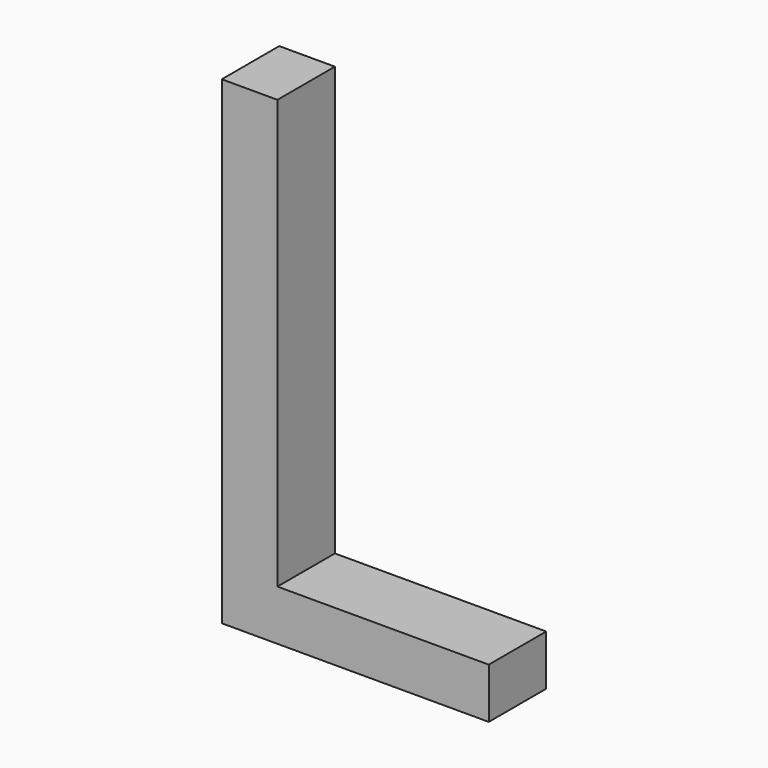
from build123d import *

# Parameters (mm, degrees)
F0_TEXT_SIZE = 237.245267878
F1_DEPTH     = 25.4


# Not quite as in the source:
# - Text() gives the source's letters only with a copy of the font that has no kerning and outlines rounded to 1/6400 em; it was checked with that copy


with BuildPart() as f1:
    # F0 (on Front) → F1 (new body)
    with BuildSketch(Plane.XZ):
        with Locations((-77.5483176112, -86.0451906919)):
            Text('L', F0_TEXT_SIZE, font='Open Sans', text_align=(TextAlign.LEFT, TextAlign.BOTTOM))
    extrude(amount=-F1_DEPTH)


solid = f1.part
